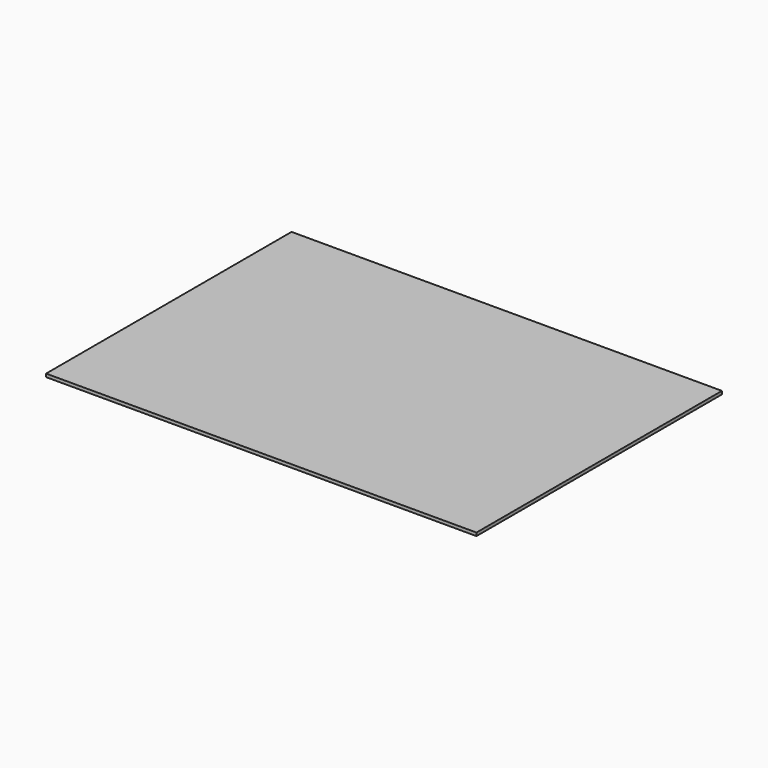
from build123d import *

# Parameters (mm, degrees)
F0_W     = 647.7
F0_H     = 461.772
F1_DEPTH = 4.7625


# Not quite as in the source:
# - a length typed as a fraction of an inch, garbled in the dataset ("3 / 203.2 mm" for 3/8 in), is restored


with BuildPart() as f1:
    # F0 (on Top) → F1 (new body)
    with BuildSketch(Plane.XY):
        with Locations((-19.7334215045, 154.33693651)):
            Rectangle(F0_W, F0_H)
    extrude(amount=-F1_DEPTH)


solid = f1.part
